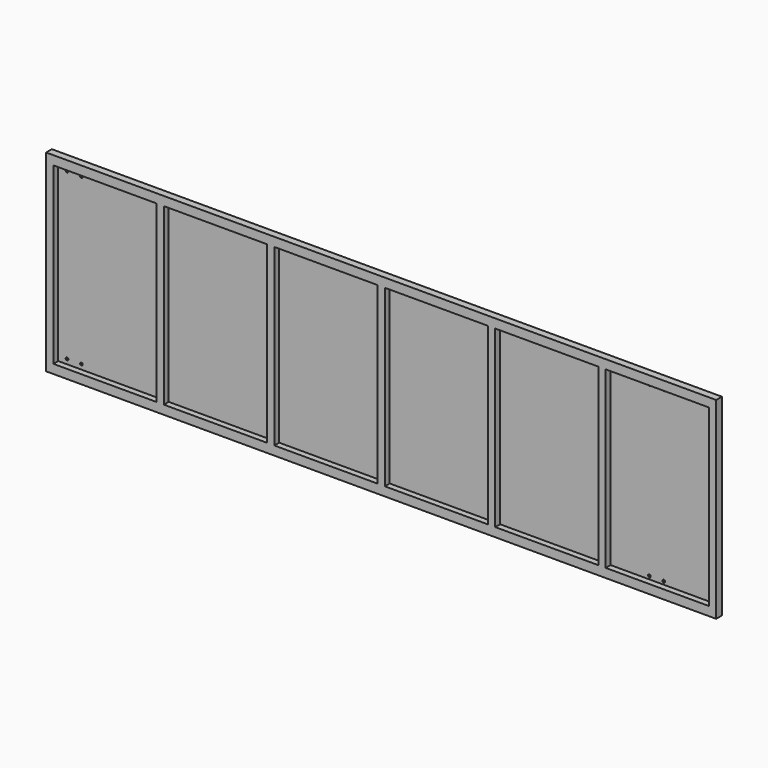
from build123d import *

# Parameters (mm, degrees)
F0_W     = 244.856
F0_H     = 414.782
F1_DEPTH = 17.018
F2_DEPTH = 2.54
F4_D     = 6.35
F4_DEPTH = 2.54
F4_TIP   = 1.9077324654


# Not quite as in the source:
# - a feature names something its author has since deleted; it is built from what else it names


with BuildPart() as f1:
    # F0 (on Front) → F1 (new body)
    with BuildSketch(Plane.XZ):
        Polygon((350.52, 228.6), (139.7, 228.6), (105.41, 228.6), (-139.7, 228.6), (-139.7, -228.6), (105.41, -228.6), (139.7, -228.6), (350.52, -228.6), (384.81, -228.6), (595.63, -228.6), (629.92, -228.6), (840.74, -228.6), (875.03, -228.6), (1085.85, -228.6), (1120.14, -228.6), (1365.25, -228.6), (1450.34, -228.6), (1450.34, 228.6), (1365.25, 228.6), (1120.14, 228.6), (1085.85, 228.6), (875.03, 228.6), (840.74, 228.6), (629.92, 228.6), (595.63, 228.6), (384.81, 228.6), align=None)
        Rectangle(F0_W, F0_H, mode=Mode.SUBTRACT)
        with Locations((262.128, 0)):
            Rectangle(F0_W, F0_H, mode=Mode.SUBTRACT)
        Polygon((629.92, 207.391), (646.684, 207.391), (646.684, -207.391), (629.92, -207.391), (401.828, -207.391), (401.828, 207.391), align=None, mode=Mode.SUBTRACT)
        Polygon((875.03, 207.391), (908.812, 207.391), (908.812, -207.391), (875.03, -207.391), (663.956, -207.391), (663.956, 207.391), align=None, mode=Mode.SUBTRACT)
        Polygon((1120.14, 207.391), (1170.94, 207.391), (1170.94, -207.391), (1120.14, -207.391), (926.084, -207.391), (926.084, 207.391), align=None, mode=Mode.SUBTRACT)
        with Locations((1310.64, 0)):
            Rectangle(F0_W, F0_H, mode=Mode.SUBTRACT)
    extrude(amount=F1_DEPTH)

    # F0 (on Front) → F2 (join)
    with BuildSketch(Plane.XZ):
        Polygon((350.52, 228.6), (139.7, 228.6), (105.41, 228.6), (-139.7, 228.6), (-139.7, -228.6), (105.41, -228.6), (139.7, -228.6), (350.52, -228.6), (384.81, -228.6), (595.63, -228.6), (629.92, -228.6), (840.74, -228.6), (875.03, -228.6), (1085.85, -228.6), (1120.14, -228.6), (1365.25, -228.6), (1450.34, -228.6), (1450.34, 228.6), (1365.25, 228.6), (1120.14, 228.6), (1085.85, 228.6), (875.03, 228.6), (840.74, 228.6), (629.92, 228.6), (595.63, 228.6), (384.81, 228.6), align=None)
        Rectangle(F0_W, F0_H, mode=Mode.SUBTRACT)
        with Locations((262.128, 0)):
            Rectangle(F0_W, F0_H, mode=Mode.SUBTRACT)
        Polygon((629.92, 207.391), (646.684, 207.391), (646.684, -207.391), (629.92, -207.391), (401.828, -207.391), (401.828, 207.391), align=None, mode=Mode.SUBTRACT)
        Polygon((875.03, 207.391), (908.812, 207.391), (908.812, -207.391), (875.03, -207.391), (663.956, -207.391), (663.956, 207.391), align=None, mode=Mode.SUBTRACT)
        Polygon((1120.14, 207.391), (1170.94, 207.391), (1170.94, -207.391), (1120.14, -207.391), (926.084, -207.391), (926.084, 207.391), align=None, mode=Mode.SUBTRACT)
        with Locations((1310.64, 0)):
            Rectangle(F0_W, F0_H, mode=Mode.SUBTRACT)
        Rectangle(F0_W, F0_H)
        with Locations((262.128, 0)):
            Rectangle(F0_W, F0_H)
        Polygon((646.684, -207.391), (646.684, 207.391), (629.92, 207.391), (401.828, 207.391), (401.828, -207.391), (629.92, -207.391), align=None)
        Polygon((908.812, -207.391), (908.812, 207.391), (875.03, 207.391), (663.956, 207.391), (663.956, -207.391), (875.03, -207.391), align=None)
        Polygon((1170.94, -207.391), (1170.94, 207.391), (1120.14, 207.391), (926.084, 207.391), (926.084, -207.391), (1120.14, -207.391), align=None)
        with Locations((1310.64, 0)):
            Rectangle(F0_W, F0_H)
    extrude(amount=F2_DEPTH)

    # F4
    with Locations(Plane(origin=(0, 0, 0), x_dir=(-1, 0, 0), z_dir=(0, 1, 0))):
        with Locations((-1314.45, 200.061827898), (-1280.31875, 200.061827898), (67.4624, 195.9268003702), (101.6, 195.9268003702), (-1314.45, -200.061827898), (-1280.31875, -200.061827898), (67.4624, -195.9268003702), (101.6, -195.9268003702)):
            Hole(F4_D / 2, depth=F4_DEPTH)
            with Locations((0, 0, -(F4_DEPTH + F4_TIP / 2))):  # 118° drill point
                Cone(0, F4_D / 2, F4_TIP, mode=Mode.SUBTRACT)


solid = f1.part
